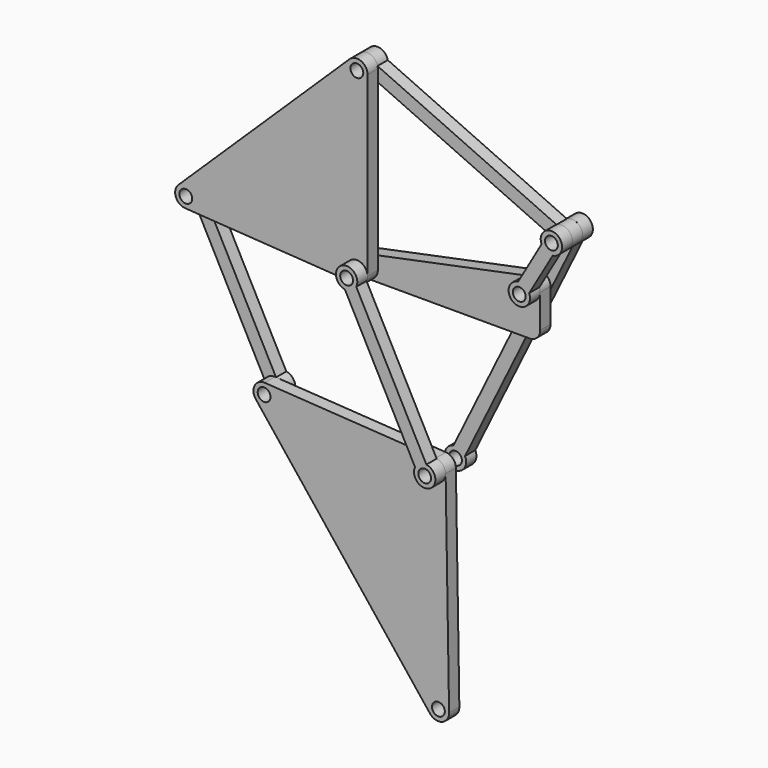
from build123d import *

# Parameters (mm, degrees)
F4_R      = 38.1
F5_DEPTH  = 76.2
F7_R      = 38.1
F8_DEPTH  = 76.2
F6_R      = 38.1
F9_DEPTH  = 76.2
F10_R     = 38.1
F11_DEPTH = 76.2
F13_R     = 38.1
F16_DEPTH = 76.2
F15_R     = 38.1
F17_DEPTH = 76.2
F14_R     = 38.1
F18_DEPTH = 76.2
F12_R     = 38.1
F19_DEPTH = 76.2


# Not quite as in the source:
# - a variable given as a bare number and used for a length is read in inches; the dataset says mm whatever the document's units were


with BuildPart() as f5:
    # F4 (on Front) → F5 (new body)
    with BuildSketch(Plane.XZ):
        with BuildLine():
            Line((-44.2566783262, 1099.6367590363), (-1060.6371400165, 111.8276987953))
            ThreePointArc((-1060.6371400165, 111.8276987953), (-1075.9648961572, 44.3376901303), (-1020.5133132963, 2.925574317))
            Line((-1020.5133132963, 2.925574317), (-4.1328516059, -63.365365442))
            ThreePointArc((-4.1328516059, -63.365365442), (43.4155152165, -46.3394328676), (63.5, 0))
            Line((63.5, 0), (63.5, 1054.1))
            ThreePointArc((63.5, 1054.1), (24.7179178561, 1112.591662114), (-44.2566783262, 1099.6367590363))
        make_face()
        with Locations((-1016.3804616903, 66.290939759)):
            Circle(F4_R, mode=Mode.SUBTRACT)
        Circle(F4_R, mode=Mode.SUBTRACT)
        with Locations((0, 1054.1)):
            Circle(F4_R, mode=Mode.SUBTRACT)
    extrude(amount=F5_DEPTH)


with BuildPart() as f8:
    # F7 (on offset) → F8 (new body)
    with BuildSketch(Plane.XZ.offset(-76.2)):
        with BuildLine():
            Line((952.4319914548, 260.3231185536), (-12.7680085452, 62.2031185536))
            ThreePointArc((-12.7680085452, 62.2031185536), (-63.1749476777, -6.4168517144), (0, -63.5))
            Line((0, -63.5), (965.2, -63.5))
            ThreePointArc((965.2, -63.5), (1010.1012806053, -44.9012806053), (1028.7, 0))
            Line((1028.7, 0), (1028.7, 198.12))
            ThreePointArc((1028.7, 198.12), (1005.3340345429, 247.3288332651), (952.4319914548, 260.3231185536))
        make_face()
        Circle(F7_R, mode=Mode.SUBTRACT)
        with Locations((965.2, 198.12)):
            Circle(F7_R, mode=Mode.SUBTRACT)
    extrude(amount=F8_DEPTH)


with BuildPart() as f9:
    # F6 (on Front) → F9 (new body)
    with BuildSketch(Plane.XZ):
        with BuildLine():
            Line((-541.1232558193, -757.1203790043), (-959.0348976054, 39.0194110198))
            ThreePointArc((-959.0348976054, 39.0194110198), (-1045.8939957148, 122.5155012014), (-1026.5043713362, 3.6031701905))
            Line((-1026.5043713362, 3.6031701905), (-608.5927295501, -792.5366198337))
            ThreePointArc((-608.5927295501, -792.5366198337), (-521.7336314407, -876.0327100153), (-541.1232558193, -757.1203790043))
        make_face()
        with Locations((-551.2471654652, -819.8081485729)):
            Circle(F6_R, mode=Mode.SUBTRACT)
        with Locations((-1016.3804616903, 66.290939759)):
            Circle(F6_R, mode=Mode.SUBTRACT)
    extrude(amount=-F9_DEPTH)


with BuildPart() as f11:
    # F10 (on Front) → F11 (new body)
    with BuildSketch(Plane.XZ):
        with BuildLine():
            Line((1125.4388332322, 583.6877524417), (62.0196468061, 1067.7313392609))
            ThreePointArc((62.0196468061, 1067.7313392609), (-57.7945210014, 1080.406716675), (30.4515867962, 998.3779140592))
            Line((30.4515867962, 998.3779140592), (1093.8707732223, 514.33432724))
            ThreePointArc((1093.8707732223, 514.33432724), (1213.6849410298, 501.6589498259), (1125.4388332322, 583.6877524417))
        make_face()
        with Locations((1155.8904200284, 527.9656665009)):
            Circle(F10_R, mode=Mode.SUBTRACT)
        with Locations((0, 1054.1)):
            Circle(F10_R, mode=Mode.SUBTRACT)
    extrude(amount=-F11_DEPTH)


with BuildPart() as f16:
    # F13 (on Front) → F16 (new body)
    with BuildSketch(Plane.XZ):
        with BuildLine():
            Line((-601.0368422679, -859.2192901941), (434.6879595358, -2167.6919965692))
            ThreePointArc((434.6879595358, -2167.6919965692), (505.8353789309, -2188.0813301248), (547.9690010872, -2127.2336671178))
            Line((547.9690010872, -2127.2336671178), (527.4441196129, -882.8029180439))
            ThreePointArc((527.4441196129, -882.8029180439), (509.88593011, -840.0049988287), (467.9505849255, -820.4760784277))
            Line((467.9505849255, -820.4760784277), (-547.2493354038, -756.4341211263))
            ThreePointArc((-547.2493354038, -756.4341211263), (-607.5092401875, -790.3661896039), (-601.0368422679, -859.2192901941))
        make_face()
        with Locations((484.4776363385, -2128.2808549481)):
            Circle(F13_R, mode=Mode.SUBTRACT)
        with Locations((-551.2471654652, -819.8081485729)):
            Circle(F13_R, mode=Mode.SUBTRACT)
        with Locations((463.9527548642, -883.8501058743)):
            Circle(F13_R, mode=Mode.SUBTRACT)
    extrude(amount=F16_DEPTH)


with BuildPart() as f17:
    # F15 (on offset) → F17 (new body)
    with BuildSketch(Plane.XZ.offset(-76.2)):
        with BuildLine():
            Line((520.5213976573, -855.0015590729), (1167.7458049756, 465.5821763151))
            ThreePointArc((1167.7458049756, 465.5821763151), (1183.836206182, 584.9856896178), (1099.3217772353, 499.1171196995))
            Line((1099.3217772353, 499.1171196995), (452.0973699169, -821.4666156885))
            ThreePointArc((452.0973699169, -821.4666156885), (436.0069687106, -940.8701289912), (520.5213976573, -855.0015590729))
        make_face()
        with Locations((463.9527548642, -883.8501058743)):
            Circle(F15_R, mode=Mode.SUBTRACT)
        with Locations((1155.8904200284, 527.9656665009)):
            Circle(F15_R, mode=Mode.SUBTRACT)
    extrude(amount=-F17_DEPTH)


with BuildPart() as f18:
    # F14 (on offset) → F18 (new body)
    with BuildSketch(Plane.XZ.offset(76.2)):
        with BuildLine():
            Line((474.0766645101, -821.1623363057), (57.345564085, -27.2715287392))
            ThreePointArc((57.345564085, -27.2715287392), (-29.5135340244, 56.2245614424), (-10.1239096459, -62.6877695686))
            Line((-10.1239096459, -62.6877695686), (406.6071907792, -856.578577135))
            ThreePointArc((406.6071907792, -856.578577135), (493.4662888886, -940.0746673166), (474.0766645101, -821.1623363057))
        make_face()
        with Locations((463.9527548642, -883.8501058743)):
            Circle(F14_R, mode=Mode.SUBTRACT)
        Circle(F14_R, mode=Mode.SUBTRACT)
    extrude(amount=F18_DEPTH)


with BuildPart() as f19:
    # F12 (on Front) → F19 (new body)
    with BuildSketch(Plane.XZ):
        with BuildLine():
            ThreePointArc((957.640822687, 261.168464203), (933.4182633286, 143.1457222499), (1023.6099559872, 223.0303801973))
            Line((1023.6099559872, 223.0303801973), (1163.4495973414, 464.9172022979))
            ThreePointArc((1163.4495973414, 464.9172022979), (1187.6721566998, 582.939944251), (1097.4804640412, 503.0552863036))
            Line((1097.4804640412, 503.0552863036), (957.640822687, 261.168464203))
        make_face()
        with Locations((965.2, 198.12)):
            Circle(F12_R, mode=Mode.SUBTRACT)
        with Locations((1155.8904200284, 527.9656665009)):
            Circle(F12_R, mode=Mode.SUBTRACT)
    extrude(amount=F19_DEPTH)


solid = Compound([f5.part, f8.part, f9.part, f11.part, f16.part, f17.part, f18.part, f19.part])
